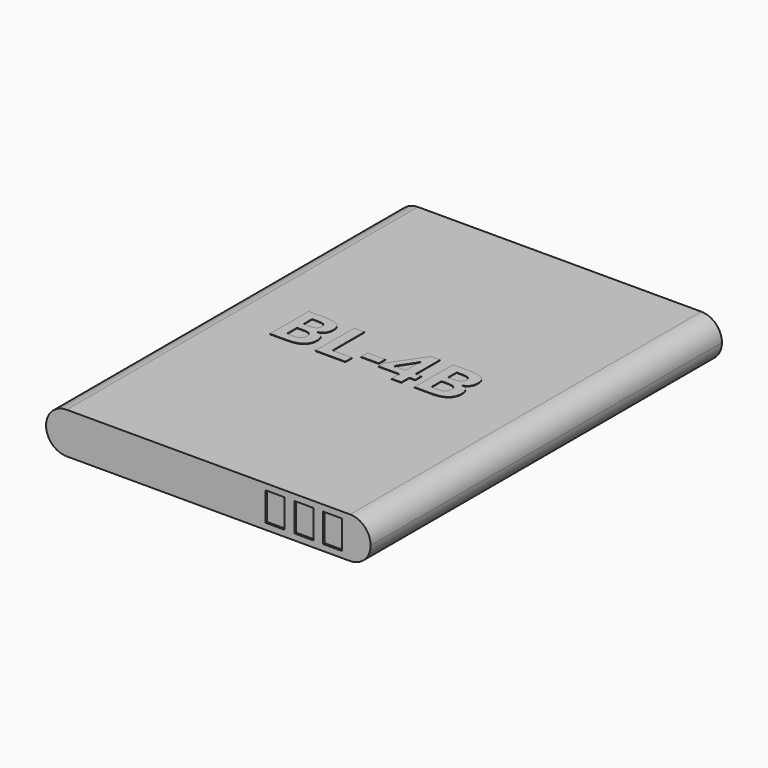
from build123d import *

# Parameters (mm, degrees)
F0_W         = 34
F0_H         = 46
F1_DEPTH     = 4.3
F2_R         = 2.14999
F3_W         = 2
F3_H         = 3
F4_DEPTH     = 2
F5_W         = 2
F5_H         = 3
F6_DEPTH     = 1.8
F7_TEXT_SIZE = 7.1087415306
F8_DEPTH     = 0.05


# Not quite as in the source:
# - a fillet or chamfer is up to 0.001 mm smaller than in the source, because OpenCascade refuses the exact size
# - Text() gives the source's letters only with a copy of the font that has no kerning and outlines rounded to 1/6400 em; it was checked with that copy


with BuildPart() as f1:
    # F0 (on Top) → F1 (new body)
    with BuildSketch(Plane.XY):
        Rectangle(F0_W, F0_H)
    extrude(amount=F1_DEPTH)

    # F2 (radius 2.15 in the source; OpenCascade refuses exactly that, so slightly less here)
    f2_edges = [f1.edges().sort_by_distance(p)[0] for p in [
        (-17, 0, 4.3),
        (17, 0, 4.3),
        (17, 0, 0),
        (-17, 0, 0),
    ]]
    fillet(f2_edges, radius=F2_R)

    # F3 (on face) → F4 (cut)
    with BuildSketch(Plane.XZ.offset(23)):
        with Locations((13, 2.15)):
            Rectangle(F3_W, F3_H)
        with Locations((10, 2.15)):
            Rectangle(F3_W, F3_H)
        with Locations((7, 2.15)):
            Rectangle(F3_W, F3_H)
    extrude(amount=-F4_DEPTH, mode=Mode.SUBTRACT)


with BuildPart() as f6:
    # F5 (on face) → F6 (new body)
    with BuildSketch(Plane.XZ.offset(21)):
        with Locations((7, 2.15)):
            Rectangle(F5_W, F5_H)
    extrude(amount=F6_DEPTH)


with BuildPart() as f6b:
    # F5 (on face) → F6, piece 2 (new body)
    with BuildSketch(Plane.XZ.offset(21)):
        with Locations((10, 2.15)):
            Rectangle(F5_W, F5_H)
    extrude(amount=F6_DEPTH)


with BuildPart() as f6c:
    # F5 (on face) → F6, piece 3 (new body)
    with BuildSketch(Plane.XZ.offset(21)):
        with Locations((13, 2.15)):
            Rectangle(F5_W, F5_H)
    extrude(amount=F6_DEPTH)


with BuildPart() as f8:
    # F7 (on face) → F8 (new body)
    with BuildSketch(Plane.XY.offset(4.3)):
        with Locations((-10.85, -2.1808316821)):
            Text('BL-4B', F7_TEXT_SIZE, font='Open Sans', font_style=FontStyle.BOLD, text_align=(TextAlign.LEFT, TextAlign.BOTTOM))
    extrude(amount=F8_DEPTH)


solid = Compound([f1.part, f6.part, f6b.part, f6c.part, f8.part])
